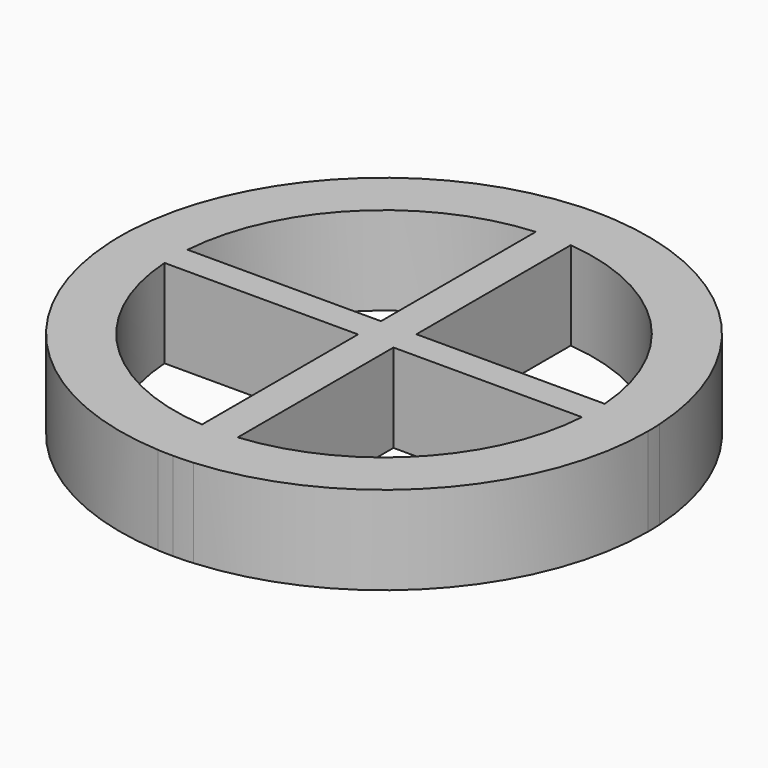
from build123d import *

# Parameters (mm, degrees)
F0_W     = 5.8146030642
F0_H     = 3.8764025085
F1_DEPTH = 25.4


with BuildPart() as f1:
    # F0 (on Top) → F1 (new body)
    with BuildSketch(Plane.XY):
        with BuildLine():
            Line((60.0847271035, 0), (75.8325080935, 0))
            ThreePointArc((75.8325080935, 0), (75.8011270946, 2.1813791382), (75.7070100699, 4.3609528802))
            Line((75.7070100699, 4.3609528802), (59.9262590279, 4.3609528802))
            ThreePointArc((59.9262590279, 4.3609528802), (60.0450970152, 2.1819155663), (60.0847271035, 0))
        make_face()
        with BuildLine():
            ThreePointArc((5.8146030642, -75.6092565428), (55.6394878556, -51.524913148), (75.8325080935, 0))
            Line((75.8325080935, 0), (60.0847271035, 0))
            ThreePointArc((60.0847271035, 0), (60.0534252964, -1.939211508), (59.9595524891, -3.8764025085))
            ThreePointArc((59.9595524891, -3.8764025085), (43.1682524028, -41.793258016), (5.8146030642, -59.8027158439))
            Line((5.8146030642, -59.8027158439), (5.8146030642, -75.6092565428))
        make_face()
        with BuildLine():
            Line((59.9262590279, 4.3609528802), (75.7070100699, 4.3609528802))
            ThreePointArc((75.7070100699, 4.3609528802), (54.1343102449, 53.1041028364), (5.8146030642, 75.6092565428))
            Line((5.8146030642, 75.6092565428), (5.8146030642, 59.8027158439))
            ThreePointArc((5.8146030642, 59.8027158439), (42.9989826308, 41.9673911962), (59.9262590279, 4.3609528802))
        make_face()
        with BuildLine():
            ThreePointArc((0, -75.8325080935), (2.9094436775, -75.7766746515), (5.8146030642, -75.6092565428))
            Line((5.8146030642, -75.6092565428), (5.8146030642, -59.8027158439))
            ThreePointArc((5.8146030642, -59.8027158439), (2.9107189466, -60.0141828763), (0, -60.0847271035))
            Line((0, -60.0847271035), (0, -75.8325080935))
        make_face()
        with BuildLine():
            Line((5.8146030642, 0), (60.0847271035, 0))
            ThreePointArc((60.0847271035, 0), (60.0450970152, 2.1819155663), (59.9262590279, 4.3609528802))
            Line((59.9262590279, 4.3609528802), (5.8146030642, 4.3609528802))
            Line((5.8146030642, 4.3609528802), (0, 4.3609528802))
            Line((0, 4.3609528802), (0, 0))
            Line((0, 0), (5.8146030642, 0))
        make_face()
        with BuildLine():
            ThreePointArc((59.9595524891, -3.8764025085), (60.0534252964, -1.939211508), (60.0847271035, 0))
            Line((60.0847271035, 0), (5.8146030642, 0))
            Line((5.8146030642, 0), (5.8146030642, -3.8764025085))
            Line((5.8146030642, -3.8764025085), (59.9595524891, -3.8764025085))
        make_face()
        with BuildLine():
            Line((5.8146030642, 59.8027158439), (5.8146030642, 75.6092565428))
            ThreePointArc((5.8146030642, 75.6092565428), (2.9094436775, 75.7766746515), (0, 75.8325080935))
            Line((0, 75.8325080935), (0, 60.0847271035))
            ThreePointArc((0, 60.0847271035), (2.9107189466, 60.0141828763), (5.8146030642, 59.8027158439))
        make_face()
        with BuildLine():
            ThreePointArc((-4.3609519489, -75.7070101236), (-2.1813786719, -75.801127108), (0, -75.8325080935))
            Line((0, -75.8325080935), (0, -60.0847271035))
            ThreePointArc((0, -60.0847271035), (-2.1819150998, -60.0450970321), (-4.3609519489, -59.9262590956))
            Line((-4.3609519489, -59.9262590956), (-4.3609519489, -75.7070101236))
        make_face()
        with BuildLine():
            ThreePointArc((0, -60.0847271035), (2.9107189466, -60.0141828763), (5.8146030642, -59.8027158439))
            Line((5.8146030642, -59.8027158439), (5.8146030642, -3.8764025085))
            Line((5.8146030642, -3.8764025085), (0, -3.8764025085))
            Line((0, -3.8764025085), (0, -60.0847271035))
        make_face()
        with Locations((2.9073015321, -1.9382012542)):
            Rectangle(F0_W, F0_H)
        with BuildLine():
            Line((0, 60.0847271035), (0, 75.8325080935))
            ThreePointArc((0, 75.8325080935), (-2.1813786719, 75.801127108), (-4.3609519489, 75.7070101236))
            Line((-4.3609519489, 75.7070101236), (-4.3609519489, 59.9262590956))
            ThreePointArc((-4.3609519489, 59.9262590956), (-2.1819150998, 60.0450970321), (0, 60.0847271035))
        make_face()
        with BuildLine():
            Line((5.8146030642, 4.3609528802), (5.8146030642, 59.8027158439))
            ThreePointArc((5.8146030642, 59.8027158439), (2.9107189466, 60.0141828763), (0, 60.0847271035))
            Line((0, 60.0847271035), (0, 4.3609528802))
            Line((0, 4.3609528802), (5.8146030642, 4.3609528802))
        make_face()
        with BuildLine():
            ThreePointArc((-75.733366407, -3.8764025085), (-53.7929735729, -53.4498388953), (-4.3609519489, -75.7070101236))
            Line((-4.3609519489, -75.7070101236), (-4.3609519489, -59.9262590956))
            ThreePointArc((-4.3609519489, -59.9262590956), (-42.6576889746, -42.3142529468), (-59.9595524891, -3.8764025085))
            Line((-59.9595524891, -3.8764025085), (-75.733366407, -3.8764025085))
        make_face()
        with BuildLine():
            ThreePointArc((-4.3609519489, -59.9262590956), (-2.1819150998, -60.0450970321), (0, -60.0847271035))
            Line((0, -60.0847271035), (0, -3.8764025085))
            Line((0, -3.8764025085), (-4.3609519489, -3.8764025085))
            Line((-4.3609519489, -3.8764025085), (-4.3609519489, -59.9262590956))
        make_face()
        with BuildLine():
            Line((0, -3.8764025085), (0, 0))
            Line((0, 0), (0, 4.3609528802))
            Line((0, 4.3609528802), (0, 60.0847271035))
            ThreePointArc((0, 60.0847271035), (-2.1819150998, 60.0450970321), (-4.3609519489, 59.9262590956))
            Line((-4.3609519489, 59.9262590956), (-4.3609519489, 4.3609528802))
            Line((-4.3609519489, 4.3609528802), (-4.3609519489, 0))
            Line((-4.3609519489, 0), (-4.3609519489, -3.8764025085))
            Line((-4.3609519489, -3.8764025085), (0, -3.8764025085))
        make_face()
        with BuildLine():
            Line((-4.3609519489, 59.9262590956), (-4.3609519489, 75.7070101236))
            ThreePointArc((-4.3609519489, 75.7070101236), (-53.6216803775, 53.6216810371), (-75.7070100699, 4.3609528802))
            Line((-75.7070100699, 4.3609528802), (-59.9262590279, 4.3609528802))
            ThreePointArc((-59.9262590279, 4.3609528802), (-42.4863176505, 42.4863183108), (-4.3609519489, 59.9262590956))
        make_face()
        with BuildLine():
            ThreePointArc((-75.8325080935, 0), (-75.8077186201, -1.938835055), (-75.733366407, -3.8764025085))
            Line((-75.733366407, -3.8764025085), (-59.9595524891, -3.8764025085))
            ThreePointArc((-59.9595524891, -3.8764025085), (-60.0534252964, -1.939211508), (-60.0847271035, 0))
            Line((-60.0847271035, 0), (-75.8325080935, 0))
        make_face()
        with BuildLine():
            Line((-59.9262590279, 4.3609528802), (-75.7070100699, 4.3609528802))
            ThreePointArc((-75.7070100699, 4.3609528802), (-75.8011270946, 2.1813791382), (-75.8325080935, 0))
            Line((-75.8325080935, 0), (-60.0847271035, 0))
            ThreePointArc((-60.0847271035, 0), (-60.0450970152, 2.1819155663), (-59.9262590279, 4.3609528802))
        make_face()
        with BuildLine():
            ThreePointArc((-60.0847271035, 0), (-60.0534252964, -1.939211508), (-59.9595524891, -3.8764025085))
            Line((-59.9595524891, -3.8764025085), (-4.3609519489, -3.8764025085))
            Line((-4.3609519489, -3.8764025085), (-4.3609519489, 0))
            Line((-4.3609519489, 0), (-60.0847271035, 0))
        make_face()
        with BuildLine():
            Line((-4.3609519489, 4.3609528802), (-59.9262590279, 4.3609528802))
            ThreePointArc((-59.9262590279, 4.3609528802), (-60.0450970152, 2.1819155663), (-60.0847271035, 0))
            Line((-60.0847271035, 0), (-4.3609519489, 0))
            Line((-4.3609519489, 0), (-4.3609519489, 4.3609528802))
        make_face()
    extrude(amount=F1_DEPTH)


solid = f1.part
